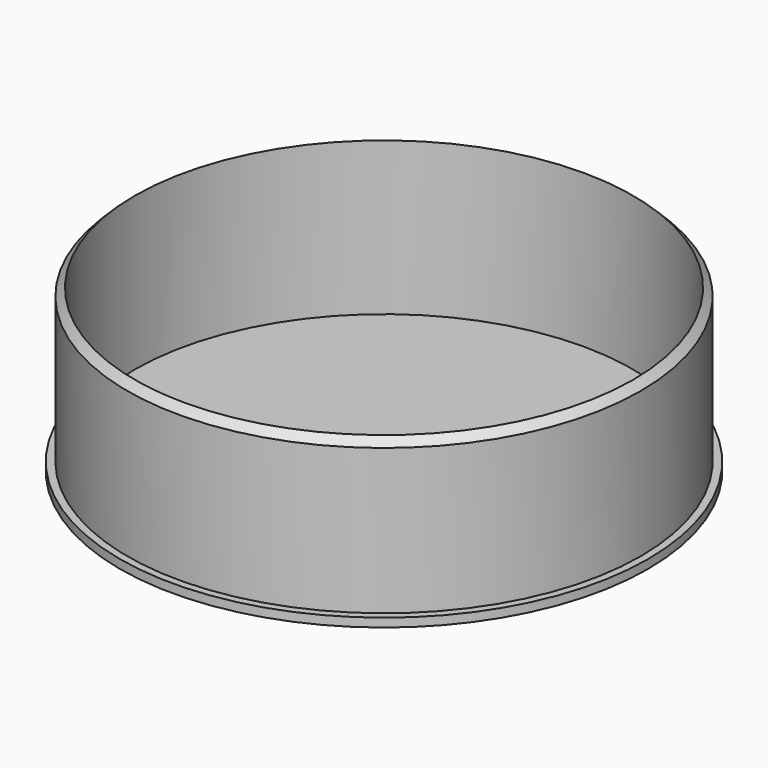
from build123d import *

# Parameters (mm, degrees)
F0_R     = 20.6375
F0_R_2   = 20.0375
F1_DEPTH = 12.7
F2_R     = 21.2375
F3_DEPTH = 0.7


# Not quite as in the source:
# - a fillet or chamfer that OpenCascade refuses, or shapes differently, is made with other operations: its cross-section is extruded or revolved along the edge and cut away or added


with BuildPart() as f1:
    # F0 (on Top) → F1 (new body)
    with BuildSketch(Plane.XY):
        Circle(F0_R)
        Circle(F0_R_2, mode=Mode.SUBTRACT)
    extrude(amount=F1_DEPTH)

    # F2 (on Top) → F3 (join)
    with BuildSketch(Plane.XY):
        Circle(F2_R)
    extrude(amount=-F3_DEPTH)

    # F4: chamfer of 1 on 1 edges, made by hand

    # F4_s1 → F4_t2 (revolve, cut)
    with BuildSketch(Plane.XZ):
        Polygon((20.6375, 11.7), (19.6375, 12.7), (20.6375, 12.7), align=None)
    revolve(axis=Axis((0, 0, 12.7), (0, 0, 1)), mode=Mode.SUBTRACT)


solid = f1.part
